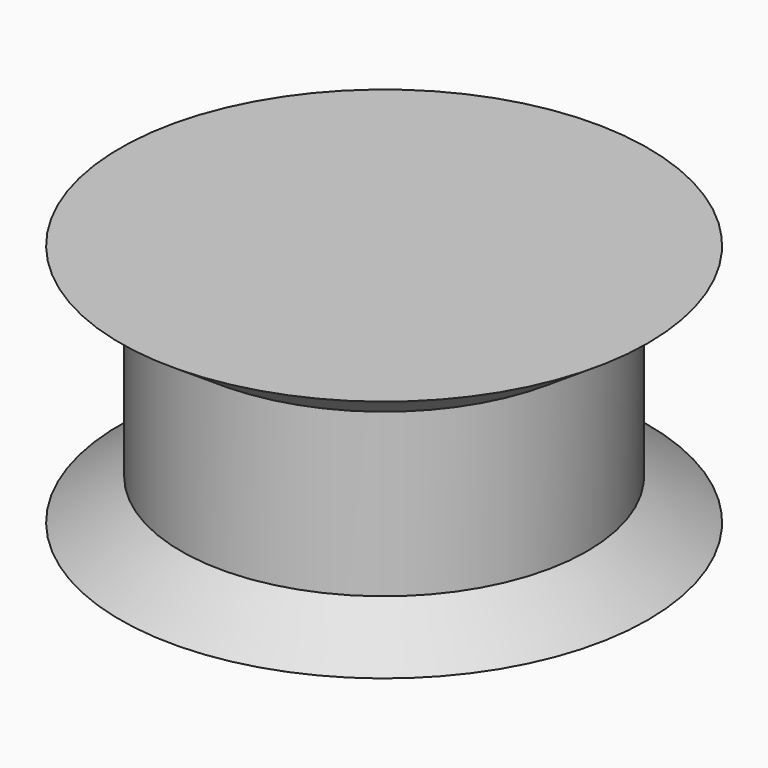
from build123d import *

# Parameters (mm, degrees)
F0_R     = 2.5
F1_DEPTH = 3
F2_START = -2.5
F0_R_2   = 3.25
F2_DEPTH = 0.5
F3_DEPTH = 0.5
F4_SIZE2 = 0.74999
F4_SIZE  = 0.49999
F5_SIZE2 = 0.49999
F5_SIZE  = 0.74999


# Not quite as in the source:
# - a fillet or chamfer is up to 0.001 mm smaller than in the source, because OpenCascade refuses the exact size


with BuildPart() as f1:
    # F0 (on Top) → F1 (new body)
    with BuildSketch(Plane.XY):
        Circle(F0_R)
    extrude(amount=-F1_DEPTH)

    # F0 (on Top) → F2 (join)
    with BuildSketch(Plane.XY.offset(F2_START)):
        Circle(F0_R_2)
        Circle(F0_R, mode=Mode.SUBTRACT)
    extrude(amount=-F2_DEPTH)

    # F0 (on Top) → F3 (join)
    with BuildSketch(Plane.XY):
        Circle(F0_R_2)
        Circle(F0_R, mode=Mode.SUBTRACT)
    extrude(amount=-F3_DEPTH)

    # F4 (size 0.5 and 0.75 in the source; OpenCascade refuses exactly that, so slightly less here)
    f4_edges = [f1.edges().sort_by_distance(p)[0] for p in [
        (-3.25, 0, -0.5),
    ]]
    f4_side = f1.faces().sort_by_distance((-3.25, 0, -0.25))[0]
    chamfer(f4_edges, length=F4_SIZE, length2=F4_SIZE2, reference=f4_side)

    # F5 (size 0.75 and 0.5 in the source; OpenCascade refuses exactly that, so slightly less here)
    f5_edges = [f1.edges().sort_by_distance(p)[0] for p in [
        (-3.25, 0, -2.5),
    ]]
    f5_side = f1.faces().sort_by_distance((-3.158076, 0, -2.5))[0]
    chamfer(f5_edges, length=F5_SIZE, length2=F5_SIZE2, reference=f5_side)


solid = f1.part
